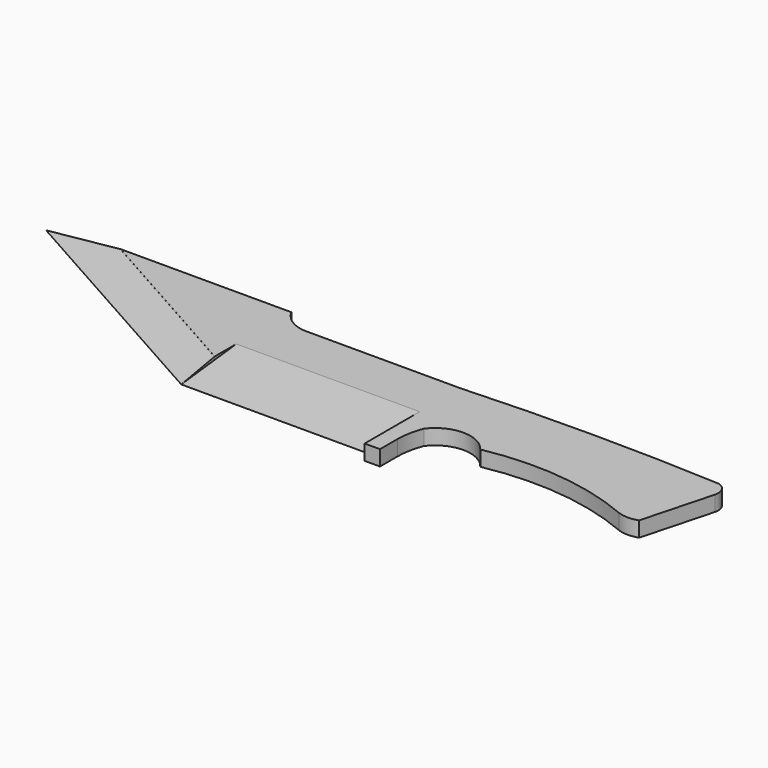
from build123d import *

# Parameters (mm, degrees)
F1_DEPTH    = 6.35
F2_DEPTH    = 6.35
F3_T1_DEPTH = 195.9699169872
F4_DEPTH    = 6.35
F5_SIZE2    = 3.17499
F5_SIZE     = 28.57499
F5_2_SIZE2  = 3.17499
F5_2_SIZE   = 28.57499


# Not quite as in the source:
# - a fillet or chamfer that OpenCascade refuses, or shapes differently, is made with other operations: its cross-section is extruded or revolved along the edge and cut away or added
# - a fillet or chamfer is up to 0.001 mm smaller than in the source, because OpenCascade refuses the exact size


with BuildPart() as f1:
    # F0 (on Top) → F1 (new body)
    with BuildSketch(Plane.XY):
        with BuildLine():
            Line((31.9449827075, -10.0934877992), (31.9449827075, -28.575))
            Line((31.9449827075, -28.575), (38.3159667253, -28.575))
            Line((38.3159667253, -28.575), (38.3159667253, -19.608527422))
            ThreePointArc((38.3159667253, -19.608527422), (38.8553616261, -13.9065356822), (40.4544100165, -8.4068356082))
            ThreePointArc((40.4544100165, -8.4068356082), (52.1485507488, -2.5894110081), (63.8426914811, -8.4068356082))
            ThreePointArc((63.8426914811, -8.4068356082), (95.8112011226, -7.0427415694), (126.7784386873, -15.0973401847))
            ThreePointArc((126.7784386873, -15.0973401847), (130.9749132386, -15.8486915066), (135.1713877899, -15.0973401847))
            Line((135.1713877899, -15.0973401847), (143.0604755878, 14.3419522792))
            ThreePointArc((143.0604755878, 14.3419522792), (142.541612074, 18.5032028423), (139.2677277327, 21.1236812174))
            ThreePointArc((139.2677277327, 21.1236812174), (85.6063552201, 22.499320446), (31.9449827075, 21.1236812174))
            Line((31.9449827075, 21.1236812174), (-30.4647367448, 21.1236812174))
            ThreePointArc((-30.4647367448, 21.1236812174), (-38.4526509093, 22.7886386215), (-44.2056395113, 28.575))
            Line((-44.2056395113, 28.575), (-115.1673197746, 28.575))
            Line((-115.1673197746, 28.575), (-44.2056395113, -11.245172738))
            Line((-44.2056395113, -11.245172738), (-44.2056395113, 0))
            Line((-44.2056395113, 0), (31.9449827075, 0))
            Line((31.9449827075, 0), (31.9449827075, -10.0934877992))
        make_face()
    extrude(amount=F1_DEPTH)


with BuildPart() as f2:
    # F0 (on Top) → F2 (new body)
    with BuildSketch(Plane.XY):
        Polygon((-146.05, 28.575), (-44.2056395113, -28.575), (-44.2056395113, -11.245172738), (-115.1673197746, 28.575), align=None)
    extrude(amount=F2_DEPTH)

    # F3: chamfer of 3.175 x 15.24 on 2 edges, made by hand

    # F3_s2 → F3_t1 (cut)
    with BuildSketch(Plane(origin=(-157.7971410428, 88.547923197, 0), x_dir=(0, 0, 1), z_dir=(0.8720780049, -0.4893668903, 0))):
        Polygon((3.175, 46.5524053311), (6.35, 31.3124053311), (6.35, 46.5524053311), align=None)
        Polygon((3.175, 46.5524053311), (0, 31.3124053311), (0, 46.5524053311), align=None)
    extrude(amount=F3_T1_DEPTH, mode=Mode.SUBTRACT)


with BuildPart() as f4:
    # F0 (on Top) → F4 (new body)
    with BuildSketch(Plane.XY):
        Polygon((-44.2056395113, -11.245172738), (-44.2056395113, -28.575), (31.9449827075, -28.575), (31.9449827075, -10.0934877992), (31.9449827075, 0), (-44.2056395113, 0), align=None)
    extrude(amount=F4_DEPTH)

    # F5 (size 28.575 and 3.175 in the source; OpenCascade refuses exactly that, so slightly less here)
    f5_edges = [f4.edges().sort_by_distance(p)[0] for p in [
        (-6.130328, -28.575, 6.35),
    ]]
    f5_side = f4.faces().sort_by_distance((-6.130328, -14.2875, 6.35))[0]
    chamfer(f5_edges, length=F5_SIZE, length2=F5_SIZE2, reference=f5_side)

    # F5#2 (size 28.575 and 3.175 in the source; OpenCascade refuses exactly that, so slightly less here)
    f5_2_edges = [f4.edges().sort_by_distance(p)[0] for p in [
        (-6.130328, -28.575, 0),
    ]]
    f5_2_side = f4.faces().sort_by_distance((-6.130328, -14.2875, 0))[0]
    chamfer(f5_2_edges, length=F5_2_SIZE, length2=F5_2_SIZE2, reference=f5_2_side)


solid = Compound([f1.part, f2.part, f4.part])
